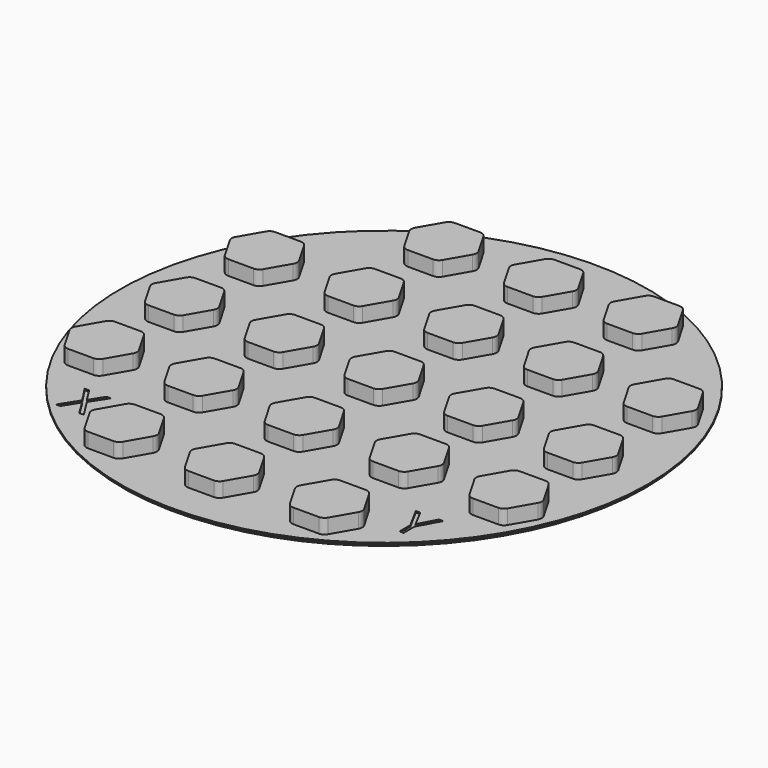
from build123d import *

# Parameters (mm, degrees)
F0_R         = 90
F1_DEPTH     = 1.5
F3_DEPTH     = 5
F4_R         = 2.5
F5_TEXT_SIZE = 20.8333333333
F6_DEPTH     = 0.5
F7_TEXT_SIZE = 16.6666666667
F8_DEPTH     = 0.5
F9_SIZE      = 1


# Not quite as in the source:
# - Text() gives the source's letters only with a copy of the font that has no kerning and outlines rounded to 1/6400 em; it was checked with that copy


with BuildPart() as f1:
    # F0 (on Top) → F1 (new body)
    with BuildSketch(Plane.XY):
        Circle(F0_R)
    extrude(amount=F1_DEPTH)

    # F2 (on face) → F3 (join)
    with BuildSketch(Plane.XY.offset(1.5)):
        Polygon((5.7735026919, 10), (-5.7735026919, 10), (-11.5470053838, 0), (-5.7735026919, -10), (5.7735026919, -10), (11.5470053838, 0), align=None)
        Polygon((5.7735026919, 24), (11.5470053838, 34), (5.7735026919, 44), (-5.7735026919, 44), (-11.5470053838, 34), (-5.7735026919, 24), align=None)
        Polygon((5.7735026919, 58), (11.5470053838, 68), (5.7735026919, 78), (-5.7735026919, 78), (-11.5470053838, 68), (-5.7735026919, 58), align=None)
        Polygon((39.7735026919, -10), (45.5470053838, 0), (39.7735026919, 10), (28.2264973081, 10), (22.4529946162, 0), (28.2264973081, -10), align=None)
        Polygon((39.7735026919, 24), (45.5470053838, 34), (39.7735026919, 44), (28.2264973081, 44), (22.4529946162, 34), (28.2264973081, 24), align=None)
        Polygon((39.7735026919, 58), (45.5470053838, 68), (39.7735026919, 78), (28.2264973081, 78), (22.4529946162, 68), (28.2264973081, 58), align=None)
        Polygon((73.7735026919, -10), (79.5470053838, 0), (73.7735026919, 10), (62.2264973081, 10), (56.4529946162, 0), (62.2264973081, -10), align=None)
        Polygon((73.7735026919, 24), (79.5470053838, 34), (73.7735026919, 44), (62.2264973081, 44), (56.4529946162, 34), (62.2264973081, 24), align=None)
        Polygon((5.7735026919, -44), (11.5470053838, -34), (5.7735026919, -24), (-5.7735026919, -24), (-11.5470053838, -34), (-5.7735026919, -44), align=None)
        Polygon((5.7735026919, -58), (-5.7735026919, -58), (-11.5470053838, -68), (-5.7735026919, -78), (5.7735026919, -78), (11.5470053838, -68), align=None)
        Polygon((-28.2264973081, 10), (-39.7735026919, 10), (-45.5470053838, 0), (-39.7735026919, -10), (-28.2264973081, -10), (-22.4529946162, 0), align=None)
        Polygon((-62.2264973081, -10), (-56.4529946162, 0), (-62.2264973081, 10), (-73.7735026919, 10), (-79.5470053838, 0), (-73.7735026919, -10), align=None)
        Polygon((-40.7735026919, -43), (-29.2264973081, -43), (-23.4529946162, -33), (-29.2264973081, -23), (-40.7735026919, -23), (-46.5470053838, -33), align=None)
        Polygon((-57.4529946162, -33), (-63.2264973081, -23), (-74.7735026919, -23), (-80.5470053838, -33), (-74.7735026919, -43), (-63.2264973081, -43), align=None)
        Polygon((-23.4529946162, -67), (-29.2264973081, -57), (-40.7735026919, -57), (-46.5470053838, -67), (-40.7735026919, -77), (-29.2264973081, -77), align=None)
        Polygon((-39.7735026919, 24), (-28.2264973081, 24), (-22.4529946162, 34), (-28.2264973081, 44), (-39.7735026919, 44), (-45.5470053838, 34), align=None)
        Polygon((-22.4529946162, 68), (-28.2264973081, 78), (-39.7735026919, 78), (-45.5470053838, 68), (-39.7735026919, 58), (-28.2264973081, 58), align=None)
        Polygon((-56.4529946162, 34), (-62.2264973081, 44), (-73.7735026919, 44), (-79.5470053838, 34), (-73.7735026919, 24), (-62.2264973081, 24), align=None)
        Polygon((57.4529946162, -33), (63.2264973081, -43), (74.7735026919, -43), (80.5470053838, -33), (74.7735026919, -23), (63.2264973081, -23), align=None)
        Polygon((23.4529946162, -67), (29.2264973081, -77), (40.7735026919, -77), (46.5470053838, -67), (40.7735026919, -57), (29.2264973081, -57), align=None)
        Polygon((23.4529946162, -33), (29.2264973081, -43), (40.7735026919, -43), (46.5470053838, -33), (40.7735026919, -23), (29.2264973081, -23), align=None)
    extrude(amount=F3_DEPTH)

    # F4
    f4_edges = [f1.edges().sort_by_distance(p)[0] for p in [
        (-40.773503, -77, 4),
        (-29.226497, -77, 4),
        (-23.452995, -67, 4),
        (-46.547005, -67, 4),
        (-40.773503, -57, 4),
        (-29.226497, -57, 4),
        (-5.773503, -78, 4),
        (5.773503, -78, 4),
        (11.547005, -68, 4),
        (-11.547005, -68, 4),
        (-5.773503, -58, 4),
        (5.773503, -58, 4),
        (23.452995, -67, 4),
        (29.226497, -57, 4),
        (40.773503, -57, 4),
        (29.226497, -77, 4),
        (46.547005, -67, 4),
        (40.773503, -77, 4),
        (-74.773503, -43, 4),
        (-63.226497, -43, 4),
        (-57.452995, -33, 4),
        (-63.226497, -23, 4),
        (-74.773503, -23, 4),
        (-80.547005, -33, 4),
        (-40.773503, -23, 4),
        (-46.547005, -33, 4),
        (-40.773503, -43, 4),
        (-29.226497, -43, 4),
        (-23.452995, -33, 4),
        (-29.226497, -23, 4),
        (-11.547005, -34, 4),
        (-5.773503, -24, 4),
        (-5.773503, -44, 4),
        (5.773503, -44, 4),
        (11.547005, -34, 4),
        (5.773503, -24, 4),
        (23.452995, -33, 4),
        (29.226497, -43, 4),
        (46.547005, -33, 4),
        (40.773503, -23, 4),
        (29.226497, -23, 4),
        (40.773503, -43, 4),
        (63.226497, -43, 4),
        (74.773503, -43, 4),
        (80.547005, -33, 4),
        (74.773503, -23, 4),
        (63.226497, -23, 4),
        (57.452995, -33, 4),
        (73.773503, -10, 4),
        (62.226497, -10, 4),
        (79.547005, 0, 4),
        (56.452995, 0, 4),
        (62.226497, 10, 4),
        (73.773503, 10, 4),
        (39.773503, 10, 4),
        (28.226497, 10, 4),
        (22.452995, 0, 4),
        (28.226497, -10, 4),
        (39.773503, -10, 4),
        (45.547005, 0, 4),
        (5.773503, -10, 4),
        (11.547005, 0, 4),
        (-5.773503, -10, 4),
        (-11.547005, 0, 4),
        (-5.773503, 10, 4),
        (5.773503, 10, 4),
        (-39.773503, 10, 4),
        (-45.547005, 0, 4),
        (-39.773503, -10, 4),
        (-28.226497, 10, 4),
        (-22.452995, 0, 4),
        (-28.226497, -10, 4),
        (-73.773503, -10, 4),
        (-62.226497, -10, 4),
        (-56.452995, 0, 4),
        (-62.226497, 10, 4),
        (-73.773503, 10, 4),
        (-79.547005, 0, 4),
        (-62.226497, 44, 4),
        (-73.773503, 44, 4),
        (-79.547005, 34, 4),
        (-73.773503, 24, 4),
        (-56.452995, 34, 4),
        (-62.226497, 24, 4),
        (-28.226497, 44, 4),
        (-39.773503, 44, 4),
        (-45.547005, 34, 4),
        (-39.773503, 24, 4),
        (-22.452995, 34, 4),
        (-28.226497, 24, 4),
        (5.773503, 44, 4),
        (-5.773503, 44, 4),
        (-11.547005, 34, 4),
        (-5.773503, 24, 4),
        (5.773503, 24, 4),
        (11.547005, 34, 4),
        (28.226497, 44, 4),
        (22.452995, 34, 4),
        (28.226497, 24, 4),
        (39.773503, 44, 4),
        (45.547005, 34, 4),
        (39.773503, 24, 4),
        (73.773503, 44, 4),
        (79.547005, 34, 4),
        (73.773503, 24, 4),
        (62.226497, 24, 4),
        (62.226497, 44, 4),
        (56.452995, 34, 4),
        (-28.226497, 78, 4),
        (-39.773503, 78, 4),
        (-45.547005, 68, 4),
        (-39.773503, 58, 4),
        (-22.452995, 68, 4),
        (-28.226497, 58, 4),
        (5.773503, 78, 4),
        (11.547005, 68, 4),
        (5.773503, 58, 4),
        (-5.773503, 58, 4),
        (-5.773503, 78, 4),
        (-11.547005, 68, 4),
        (39.773503, 78, 4),
        (28.226497, 78, 4),
        (22.452995, 68, 4),
        (28.226497, 58, 4),
        (45.547005, 68, 4),
        (39.773503, 58, 4),
    ]]
    fillet(f4_edges, radius=F4_R)

    # F5 (on face) → F6 (cut)
    with BuildSketch(Plane(origin=(0, 0, 0), x_dir=(1, 0, 0), z_dir=(0, 0, -1))):
        with Locations((-6.2044270833, -67.5)):
            Text('Z', F5_TEXT_SIZE, font='Open Sans', text_align=(TextAlign.LEFT, TextAlign.BOTTOM))
    extrude(amount=-F6_DEPTH, mode=Mode.SUBTRACT)

    # F7 (on face) → F8 (cut)
    with BuildSketch(Plane.XY.offset(1.5)):
        with Locations((-61.8862508283, -62.5685424949)):
            Text('X', F7_TEXT_SIZE, font='Open Sans', text_align=(TextAlign.LEFT, TextAlign.BOTTOM))
        with Locations((51.3615112449, -62.5685424949)):
            Text('Y', F7_TEXT_SIZE, font='Open Sans', text_align=(TextAlign.LEFT, TextAlign.BOTTOM))
    extrude(amount=-F8_DEPTH, mode=Mode.SUBTRACT)

    # F9
    f9_edges = [f1.edges().sort_by_distance(p)[0] for p in [
        (-90, 0, 0),
    ]]
    chamfer(f9_edges, length=F9_SIZE)


solid = f1.part
